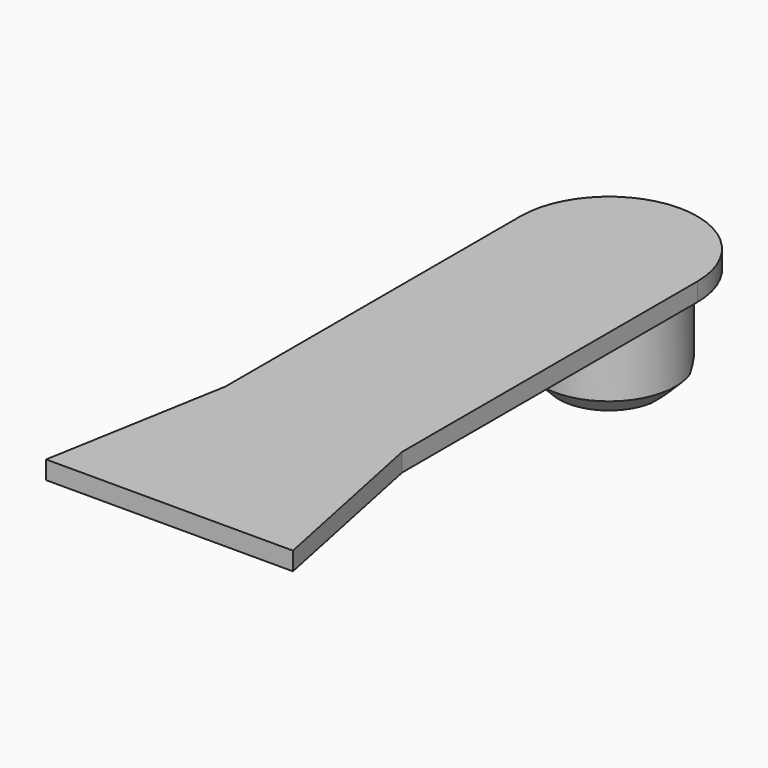
from build123d import *

# Parameters (mm, degrees)
F1_DEPTH    = 1.651
F2_R        = 6.0325
F3_DEPTH    = 8.89
F5_DEPTH    = 17.3228
F6_T2_ANGLE = 240.5568781665


# Not quite as in the source:
# - a fillet or chamfer that OpenCascade refuses, or shapes differently, is made with other operations: its cross-section is extruded or revolved along the edge and cut away or added


with BuildPart() as f1:
    # F0 (on Top) → F1 (new body)
    with BuildSketch(Plane.XY):
        with BuildLine():
            Line((-8.0826530047, 26.9640675335), (-8.0826530047, -6.4369324665))
            Line((-8.0826530047, -6.4369324665), (-11.0126939906, -23.0739324665))
            Line((-11.0126939906, -23.0739324665), (11.3393060094, -23.0739324665))
            Line((11.3393060094, -23.0739324665), (7.9193469953, -6.4369324665))
            Line((7.9193469953, -6.4369324665), (7.9193469953, 26.9640675335))
            ThreePointArc((7.9193469953, 26.9640675335), (-0.0816530047, 34.9650675335), (-8.0826530047, 26.9640675335))
        make_face()
    extrude(amount=F1_DEPTH)

    # F2 (on face) → F3 (join)
    with BuildSketch(Plane(origin=(0, 0, 0), x_dir=(1, 0, 0), z_dir=(0, 0, -1))):
        with Locations((-0.0816530047, -26.9640675335)):
            Circle(F2_R)
    extrude(amount=F3_DEPTH)

    # F4 (on face) → F5 (cut)
    with BuildSketch(Plane(origin=(-8.0826530047, 0, 0), x_dir=(0, -1, 0), z_dir=(-1, 0, 0))):
        Polygon((-24.261539802, -9.96281486), (-34.2662967741, -4.5080343261), (-34.2662967741, -10.2679394186), align=None)
    extrude(amount=-F5_DEPTH, mode=Mode.SUBTRACT)

    # F6: chamfer of 1.524 on 1 edges, made by hand

    # F6_s1 → F6_t2 (revolve, cut)
    with BuildSketch(Plane(origin=(-11.7615074362, 20.1448064433, 0), x_dir=(0, 0, 1), z_dir=(-0.5042026846, 0.8635853477, 0))):
        Polygon((-7.366, 19.5573408996), (-8.89, 18.0333408996), (-8.89, 19.5573408996), align=None)
    revolve(axis=Axis((-0.0816530047, 26.9640675335, -8.89), (0, 0, -1)), revolution_arc=F6_T2_ANGLE, mode=Mode.SUBTRACT)


solid = f1.part
